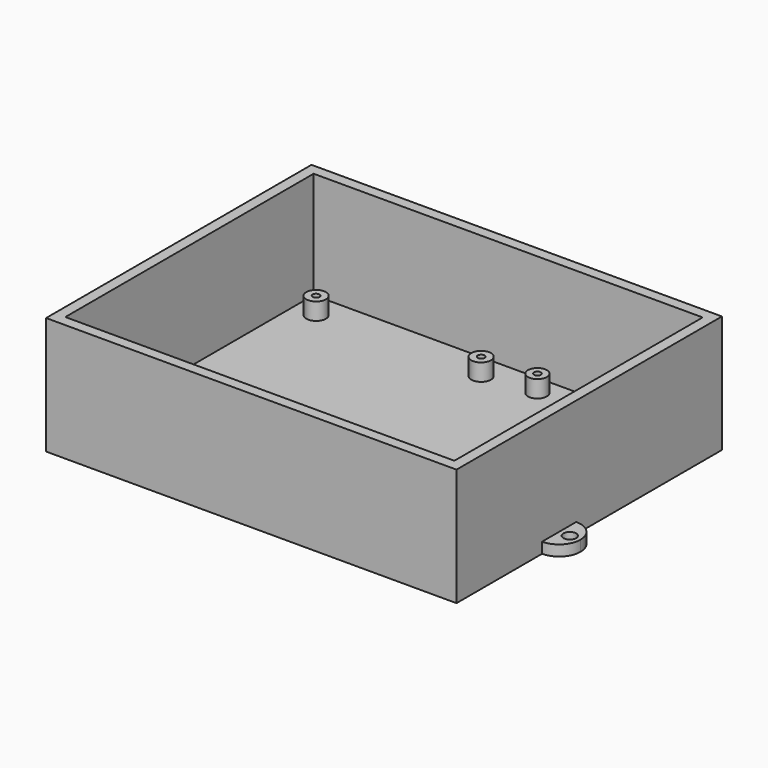
from build123d import *

# Parameters (mm, degrees)
F0_W      = 121.92
F0_H      = 98.552
F1_DEPTH  = 3.175
F2_W      = 12.7
F2_H      = 3.175
F3_DEPTH  = 6.35
F4_W      = 12.7
F4_H      = 3.175
F5_DEPTH  = 6.35
F6_R      = 6.34999
F7_R      = 1.905
F8_DEPTH  = 6.35
F9_W      = 115.57
F9_H      = 3.175
F10_DEPTH = 31.75
F11_R     = 2.921
F11_R_2   = 1.016
F12_R     = 2.794
F12_R_2   = 1.016
F13_R     = 2.921
F13_R_2   = 1.016
F14_DEPTH = 5.08


# Not quite as in the source:
# - a fillet or chamfer is up to 0.001 mm smaller than in the source, because OpenCascade refuses the exact size
# - a feature names something its author has since deleted; it is built from what else it names


with BuildPart() as f1:
    # F0 (on Top) → F1 (new body)
    with BuildSketch(Plane.XY):
        with Locations((-12.7, -8.001)):
            Rectangle(F0_W, F0_H)
    extrude(amount=F1_DEPTH)

    # F2 (on face) → F3 (join)
    with BuildSketch(Plane.YZ.offset(48.26)):
        with Locations((-19.177, 1.5875)):
            Rectangle(F2_W, F2_H)
    extrude(amount=F3_DEPTH)

    # F4 (on face) → F5 (join)
    with BuildSketch(Plane(origin=(-73.66, 0, 0), x_dir=(0, -1, 0), z_dir=(-1, 0, 0))):
        with Locations((19.177, 1.5875)):
            Rectangle(F4_W, F4_H)
    extrude(amount=F5_DEPTH)

    # F6 (radius 6.35 in the source; OpenCascade refuses exactly that, so slightly less here)
    f6_edges = [f1.edges().sort_by_distance(p)[0] for p in [
        (-80.01, -25.527, 1.5875),
        (-80.01, -12.827, 1.5875),
        (54.61, -25.527, 1.5875),
        (54.61, -12.827, 1.5875),
    ]]
    fillet(f6_edges, radius=F6_R)

    # F7 (on face) → F8 (cut)
    with BuildSketch(Plane.XY.offset(3.175)):
        with Locations((-76.835, -19.177)):
            Circle(F7_R)
        with Locations((51.435, -19.177)):
            Circle(F7_R)
    extrude(amount=-F8_DEPTH, mode=Mode.SUBTRACT)

    # F9 (on face) → F10 (join)
    with BuildSketch(Plane.XY.offset(3.175)):
        Polygon((-73.66, -57.277), (-70.485, -57.277), (-70.485, -54.102), (-70.485, 38.1), (-70.485, 41.275), (-73.66, 41.275), (-73.66, -12.827), (-73.66, -25.527), align=None)
        with Locations((-12.7, -55.6895)):
            Rectangle(F9_W, F9_H)
        with Locations((-12.7, 39.6875)):
            Rectangle(F9_W, F9_H)
        Polygon((45.085, -57.277), (48.26, -57.277), (48.26, -25.527), (48.26, -12.827), (48.26, 41.275), (45.085, 41.275), (45.085, 38.1), (45.085, -54.102), align=None)
    extrude(amount=F10_DEPTH)

    # F11 (on face) + F12 (on face) + F13 (on face) → F14 (join)
    with BuildSketch(Plane.XY.offset(3.175)):
        with Locations((-63.754, 30.607)):
            Circle(F11_R)
        with Locations((-63.754, 30.607)):
            Circle(F11_R_2, mode=Mode.SUBTRACT)
        with Locations((-14.732, -27.559)):
            Circle(F11_R)
        with Locations((-14.732, -27.559)):
            Circle(F11_R_2, mode=Mode.SUBTRACT)
        with Locations((-14.732, 30.607)):
            Circle(F11_R)
        with Locations((-14.732, 30.607)):
            Circle(F11_R_2, mode=Mode.SUBTRACT)
        with Locations((-63.754, -27.559)):
            Circle(F11_R)
        with Locations((-63.754, -27.559)):
            Circle(F11_R_2, mode=Mode.SUBTRACT)
    with BuildSketch(Plane.XY.offset(3.175)):
        with Locations((34.798, 14.605)):
            Circle(F12_R)
        with Locations((34.798, 14.605)):
            Circle(F12_R_2, mode=Mode.SUBTRACT)
        with Locations((0.762, 32.131)):
            Circle(F12_R)
        with Locations((0.762, 32.131)):
            Circle(F12_R_2, mode=Mode.SUBTRACT)
    with BuildSketch(Plane.XY.offset(3.175)):
        with Locations((40.005, -19.05)):
            Circle(F13_R)
        with Locations((40.005, -19.05)):
            Circle(F13_R_2, mode=Mode.SUBTRACT)
        with Locations((40.005, -49.022)):
            Circle(F13_R)
        with Locations((40.005, -49.022)):
            Circle(F13_R_2, mode=Mode.SUBTRACT)
        with Locations((-0.127, -49.022)):
            Circle(F13_R)
        with Locations((-0.127, -49.022)):
            Circle(F13_R_2, mode=Mode.SUBTRACT)
        with Locations((-0.127, -19.05)):
            Circle(F13_R)
        with Locations((-0.127, -19.05)):
            Circle(F13_R_2, mode=Mode.SUBTRACT)
    extrude(amount=F14_DEPTH)


solid = f1.part
